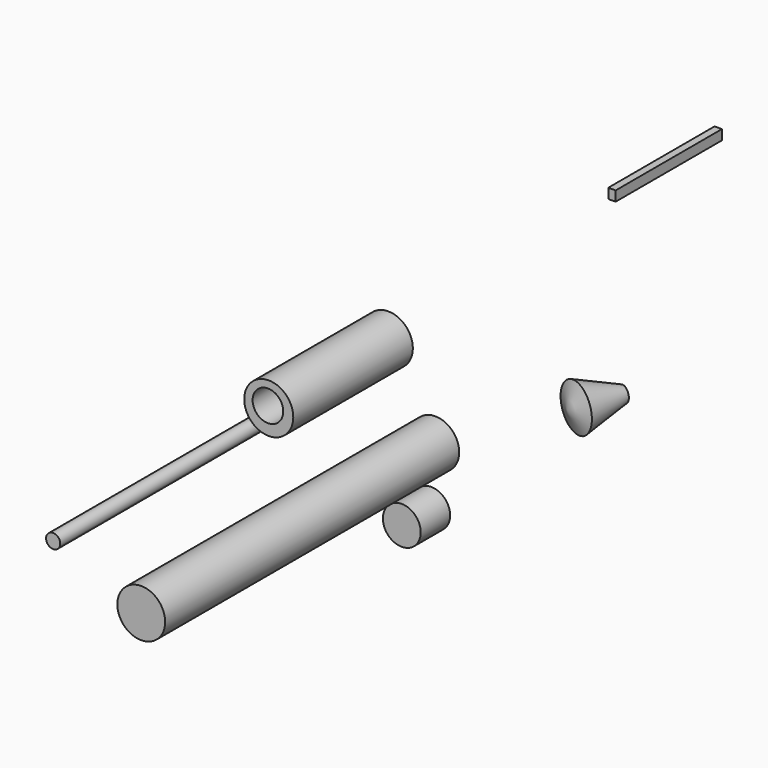
from build123d import *

# Parameters (mm, degrees)
F2_R      = 4.9560366271
F3_DEPTH  = 76.2
F4_R      = 3.9231322821
F5_DEPTH  = 7.62
F6_R      = 1.1929608885
F7_DEPTH  = 6.35
F8_W      = 27.5500733405
F8_H      = 2.0662583411
F9_DEPTH  = 1.524
F10_R     = 5.082057301
F11_DEPTH = 30.988
F13_D     = 6.35
F16_R     = 1.4700534699
F17_DEPTH = 73.66


# Not quite as in the source:
# - the program builds the solid bodies; features that only make, move or delete a surface that nothing else refers to are left out


with BuildPart() as f1:
    # F0 (on Top) → F1 (revolve)
    with BuildSketch(Plane.XY):
        Polygon((0, 19.1702581942), (0, 28.7521872672), (-1.7018, 28.7521872672), (-5.08, 19.1702581942), align=None)
    revolve(axis=Axis((-3.3909, 23.9612227307, 0), (-0.3325, -0.9431032552, 0)))


with BuildPart() as f3:
    # F2 (on Front) → F3 (new body)
    with BuildSketch(Plane.XZ):
        with Locations((-17.1269066632, -2.1915955003)):
            Circle(F2_R)
    extrude(amount=F3_DEPTH)


with BuildPart() as f5:
    # F4 (on Front) → F5 (new body)
    with BuildSketch(Plane.XZ):
        with Locations((-17.9732199758, -14.3325095996)):
            Circle(F4_R)
    extrude(amount=F5_DEPTH)


with BuildPart() as f7:
    # F6 (on Front) → F7 (new body)
    with BuildSketch(Plane.XZ):
        with Locations((-43.1825295091, 2.6402152143)):
            Circle(F6_R)
    extrude(amount=-F7_DEPTH)


with BuildPart() as f9:
    # F8 (on Right) → F9 (new body)
    with BuildSketch(Plane.YZ):
        with Locations((37.1925970539, 39.4884366542)):
            Rectangle(F8_W, F8_H)
    extrude(amount=F9_DEPTH)


with BuildPart() as f11:
    # F10 (on Front) → F11 (new body)
    with BuildSketch(Plane.XZ):
        with Locations((-26.8613211811, 13.6602437124)):
            Circle(F10_R)
    extrude(amount=F11_DEPTH)

    # F13 (through all)
    with Locations(Plane(origin=(0, 0, 0), x_dir=(1, 0, 0), z_dir=(0, 1, 0))):
        with Locations((-27.0296689123, -14.0424408019)):
            Hole(F13_D / 2)


with BuildPart() as f17:
    # F16 (on Front) → F17 (new body)
    with BuildSketch(Plane.XZ):
        with Locations((-37.4221801758, 3.328967141)):
            Circle(F16_R)
    extrude(amount=F17_DEPTH)


solid = Compound([f1.part, f3.part, f5.part, f7.part, f9.part, f11.part, f17.part])
